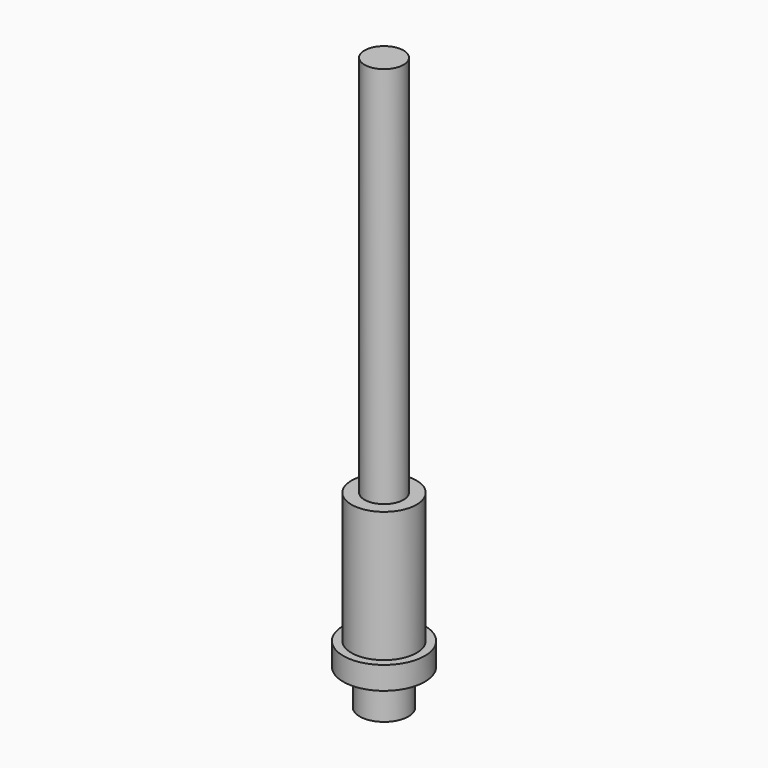
from build123d import *

# Parameters (mm, degrees)
F0_R      = 7.485
F0_R_2    = 5.985
F1_DEPTH  = 11
F2_R      = 7.485
F2_R_2    = 5.985
F3_DEPTH  = 7
F2_R_3    = 12.5
F4_DEPTH  = 7
F5_R      = 10
F6_DEPTH  = 40.05
F9_R      = 5.985
F10_DEPTH = 117.5055425


# Not quite as in the source:
# - an extrude ends at something that could not be found from the text; its depth is read off the source's solid
# - the program builds the solid bodies; features that only make, move or delete a surface that nothing else refers to are left out


with BuildPart() as f1:
    # F0 (on Top) → F1 (new body)
    with BuildSketch(Plane.XY):
        Circle(F0_R)
        Circle(F0_R_2, mode=Mode.SUBTRACT)
    extrude(amount=-F1_DEPTH)

    # F2 (on face) → F3 (join)
    with BuildSketch(Plane.XY):
        Circle(F2_R)
        Circle(F2_R_2, mode=Mode.SUBTRACT)
    extrude(amount=F3_DEPTH)

    # F2 (on face) → F4 (join)
    with BuildSketch(Plane.XY):
        Circle(F2_R_3)
    extrude(amount=F4_DEPTH)

    # F5 (on face) → F6 (join)
    with BuildSketch(Plane.XY.offset(7)):
        Circle(F5_R)
    extrude(amount=F6_DEPTH)

    # F9 (on face) → F10 (join, through all)
    with BuildSketch(Plane.XY.offset(47.05)):
        Circle(F9_R)
    extrude(amount=F10_DEPTH)


solid = f1.part
